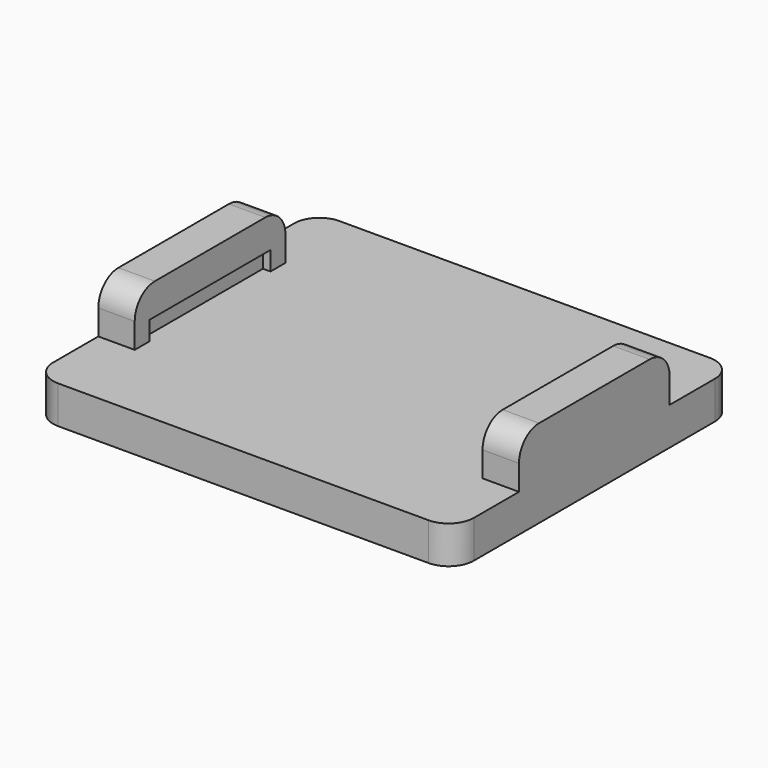
from build123d import *

# Parameters (mm, degrees)
F0_W     = 33.5
F0_H     = 28
F1_DEPTH = 3
F2_R     = 2
F3_W     = 2.9
F3_H     = 15
F4_DEPTH = 4
F5_W     = 12.03
F5_H     = 1.51
F6_DEPTH = 0.6
F7_R     = 2


# Not quite as in the source:
# - a pattern or mirror of a feature is missing from the dataset's text; its kind, count and spacing are read off the source's solid


with BuildPart() as f1:
    # F0 (on Top) → F1 (new body)
    with BuildSketch(Plane.XY):
        Rectangle(F0_W, F0_H)
    extrude(amount=F1_DEPTH)

    # F2
    f2_edges = [f1.edges().sort_by_distance(p)[0] for p in [
        (-16.75, -14, 1.5),
        (16.75, -14, 1.5),
        (16.75, 14, 1.5),
        (-16.75, 14, 1.5),
    ]]
    fillet(f2_edges, radius=F2_R)

    # F3 (on face) → F4 (join)
    with BuildSketch(Plane.XY.offset(3)):
        with Locations((15.3, 0)):
            Rectangle(F3_W, F3_H)
    f4 = extrude(amount=F4_DEPTH)

    # F4_copies: F4 across plane
    add(f4.mirror(Plane(origin=(0, 0, 0), x_dir=(0, 0, -1), z_dir=(-1, 0, 0))))

    # F5 (on face) → F6 (cut)
    with BuildSketch(Plane(origin=(13.85, 0, 0), x_dir=(0, -1, 0), z_dir=(-1, 0, 0))):
        with Locations((0, 3.755)):
            Rectangle(F5_W, F5_H)
    f6 = extrude(amount=-F6_DEPTH, mode=Mode.SUBTRACT)

    # F6_copies: F6 across plane
    add(f6.mirror(Plane(origin=(0, 0, 0), x_dir=(0, 0, -1), z_dir=(-1, 0, 0))), mode=Mode.SUBTRACT)

    # F7
    f7_edges = [f1.edges().sort_by_distance(p)[0] for p in [
        (15.3, 7.5, 7),
        (15.3, -7.5, 7),
        (-15.3, 7.5, 7),
        (-15.3, -7.5, 7),
    ]]
    fillet(f7_edges, radius=F7_R)


solid = f1.part
